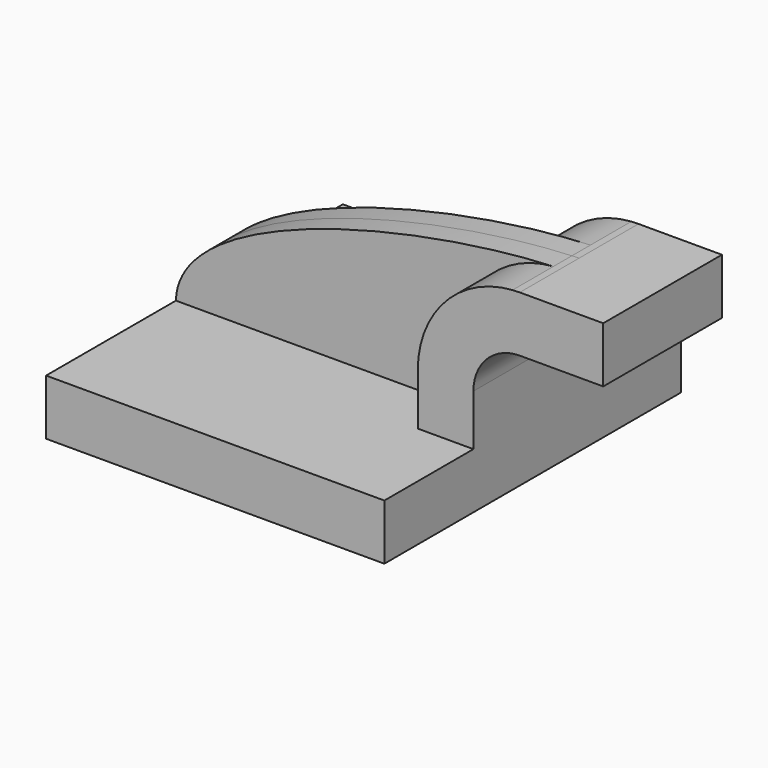
from build123d import *

# Parameters (mm, degrees)
F1_DEPTH = 63.5
F0_W     = 25.4
F0_H     = 19.05
F2_DEPTH = 25.4
F3_DEPTH = 7.9375


# Not quite as in the source:
# - the program builds the solid bodies; features that only make, move or delete a surface that nothing else refers to are left out


with BuildPart() as f1:
    # F0 (on Front) → F1 (new body, symmetric)
    with BuildSketch(Plane.XZ):
        Polygon((38.861105454, 9.525), (-57.911105454, 9.525), (-57.911105454, -9.525), (57.911105454, -9.525), (57.911105454, 9.525), align=None)
    extrude(amount=F1_DEPTH, both=True)

    # F0 (on Front) → F2 (join, symmetric)
    with BuildSketch(Plane.XZ):
        with BuildLine():
            Line((38.861105454, 27.0002), (38.861105454, 9.525))
            Line((38.861105454, 9.525), (57.911105454, 9.525))
            Line((57.911105454, 9.525), (57.911105454, 27.0002))
            ThreePointArc((57.911105454, 27.0002), (62.5607853026, 38.2255201513), (73.786105454, 42.8752))
            Line((73.786105454, 42.8752), (76.961105454, 42.8752))
            Line((76.961105454, 42.8752), (76.961105454, 61.9252))
            Line((76.961105454, 61.9252), (73.786105454, 61.9252))
            add(Edge.make_bspline(
                [(71.3194409243, 61.8379839579), (72.1527081081, 61.872613516), (72.9751435191, 61.9016976168), (73.786105454, 61.9252)],
                knots=[139.2706883943, 139.2706883943, 139.2706883943, 139.2706883943, 141.7389724845, 141.7389724845, 141.7389724845, 141.7389724845], degree=3))
            ThreePointArc((71.3194409243, 61.8379839579), (48.2331811233, 50.8078391763), (38.861105454, 27.0002))
        make_face()
        with Locations((89.661105454, 52.4002)):
            Rectangle(F0_W, F0_H)
    extrude(amount=F2_DEPTH, both=True)

    # F0 (on Front) → F3 (join, symmetric)
    with BuildSketch(Plane.XZ):
        with BuildLine():
            add(Edge.make_bspline(
                [(-57.911105454, 9.525), (-57.1981257704, 40.2751503058), (24.3030967511, 59.8840425909), (71.3194409243, 61.8379839579)],
                knots=[0, 0, 0, 0, 139.2706883943, 139.2706883943, 139.2706883943, 139.2706883943], degree=3))
            Line((-57.911105454, 9.525), (38.861105454, 9.525))
            Line((38.861105454, 9.525), (38.861105454, 27.0002))
            ThreePointArc((38.861105454, 27.0002), (48.2331811233, 50.8078391763), (71.3194409243, 61.8379839579))
        make_face()
    extrude(amount=F3_DEPTH, both=True)


solid = f1.part
